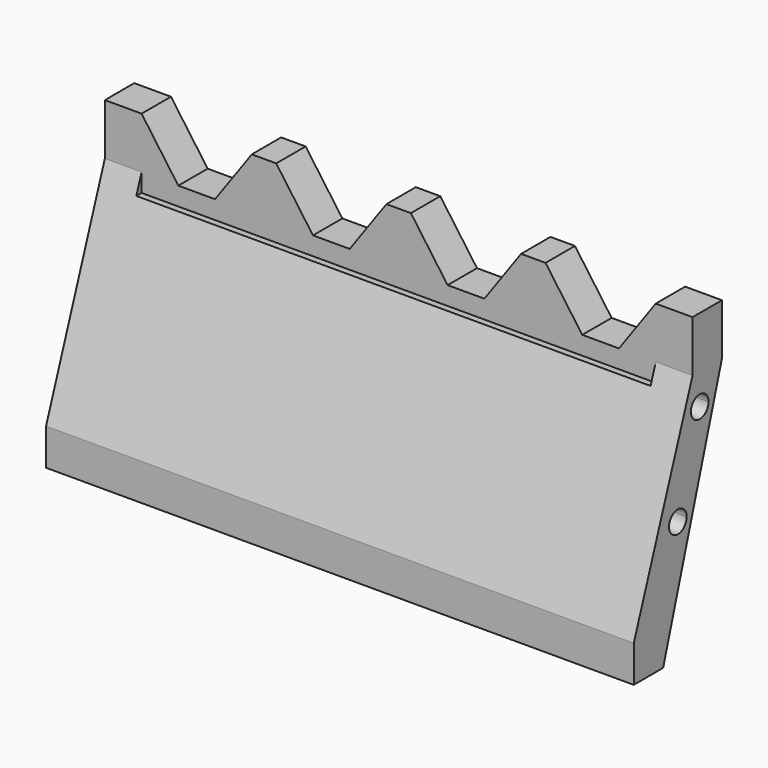
from build123d import *

# Parameters (mm, degrees)
F1_DEPTH  = 6.35
F0_W      = 88.9
F0_H      = 32.385
F2_DEPTH  = 19.05
F5_DEPTH  = 101.6
F6_DEPTH  = 12.7
F9_DEPTH  = 12.7
F11_R     = 1.905
F12_DEPTH = 5.08


# Not quite as in the source:
# - a feature names something its author has since deleted; it is built from what else it names


with BuildPart() as f1:
    # F0 (on Front) → F1 (new body)
    with BuildSketch(Plane.XZ):
        Polygon((50.8, 16.51), (50.8, 25.4), (44.4373, 25.4), (38.0873, 16.51), (31.7373, 16.51), (25.3873, 25.4), (21.1582, 25.4), (14.8082, 16.51), (8.4582, 16.51), (2.1082, 25.4), (-2.1209, 25.4), (-8.4709, 16.51), (-14.8209, 16.51), (-21.1709, 25.4), (-25.4, 25.4), (-31.75, 16.51), (-38.1, 16.51), (-44.45, 25.4), (-50.8, 25.4), (-50.8, 16.51), (-44.45, 16.51), (-44.45, 13.335), (44.45, 13.335), (44.45, 16.51), align=None)
    extrude(amount=F1_DEPTH)

    # F0 (on Front) → F2 (join)
    with BuildSketch(Plane.XZ):
        Polygon((50.8, -25.4), (50.8, 16.51), (44.45, 16.51), (44.45, 13.335), (44.45, -19.05), (-44.45, -19.05), (-44.45, 13.335), (-44.45, 16.51), (-50.8, 16.51), (-50.8, -25.4), (-44.45, -25.4), (44.45, -25.4), align=None)
        with Locations((0, -2.8575)):
            Rectangle(F0_W, F0_H)
    extrude(amount=F2_DEPTH)

    # F4 (on offset) → F5 (cut)
    with BuildSketch(Plane.YZ.offset(50.8)):
        Polygon((-12.7, -25.4), (0, -25.4), (0, 16.51), align=None)
        Polygon((-6.35, 16.51), (-6.35, 25.4), (-19.05, 25.4), (-19.05, -19.05), align=None)
    extrude(amount=-F5_DEPTH, mode=Mode.SUBTRACT)

    # F4 (on offset) → F6 (cut)
    with BuildSketch(Plane.YZ.offset(50.8)):
        with BuildLine():
            ThreePointArc((-8.972535912, -2.6218685096), (-11.3481314904, -3.892535912), (-10.077464088, -6.2681314904))
            ThreePointArc((-10.077464088, -6.2681314904), (-8.3899711651, -5.9749459284), (-7.62, -4.445))
            ThreePointArc((-7.62, -4.445), (-7.9950540716, -3.3099711651), (-8.972535912, -2.6218685096))
        make_face()
        with BuildLine():
            ThreePointArc((-2.897765424, 11.1383741007), (-3.2728194956, 12.2734029356), (-4.250301336, 12.9615055911))
            ThreePointArc((-4.250301336, 12.9615055911), (-6.6258969145, 11.6908381887), (-5.3552295121, 9.3152426102))
            ThreePointArc((-5.3552295121, 9.3152426102), (-3.6677365891, 9.6084281723), (-2.897765424, 11.1383741007))
        make_face()
    extrude(amount=-F6_DEPTH, mode=Mode.SUBTRACT)

    # F8 (on offset) → F9 (cut)
    with BuildSketch(Plane(origin=(-50.8, 0, 0), x_dir=(0, -1, 0), z_dir=(-1, 0, 0))):
        with BuildLine():
            ThreePointArc((4.2333912752, 13.0173087917), (2.9627238728, 10.6417132133), (5.3383194513, 9.3710458109))
            ThreePointArc((5.3383194513, 9.3710458109), (6.3158012916, 10.0591484663), (6.6908553632, 11.1941773013))
            ThreePointArc((6.6908553632, 11.1941773013), (5.9208841982, 12.7241232297), (4.2333912752, 13.0173087917))
        make_face()
        with BuildLine():
            ThreePointArc((8.972535912, -2.6218685096), (7.7018685096, -4.997464088), (10.077464088, -6.2681314904))
            ThreePointArc((10.077464088, -6.2681314904), (11.0549459284, -5.5800288349), (11.43, -4.445))
            ThreePointArc((11.43, -4.445), (10.6600288349, -2.9150540716), (8.972535912, -2.6218685096))
        make_face()
    extrude(amount=-F9_DEPTH, mode=Mode.SUBTRACT)

    # F11 (on offset) → F12 (cut)
    with BuildSketch(Plane(origin=(0, 0, -25.4), x_dir=(1, 0, 0), z_dir=(0, 0, -1))):
        with Locations((-38.1, 15.875)):
            Circle(F11_R)
        with Locations((-19.05, 15.875)):
            Circle(F11_R)
        with Locations((0, 15.875)):
            Circle(F11_R)
        with Locations((19.05, 15.875)):
            Circle(F11_R)
        with Locations((38.1, 15.875)):
            Circle(F11_R)
    extrude(amount=-F12_DEPTH, mode=Mode.SUBTRACT)


solid = f1.part
